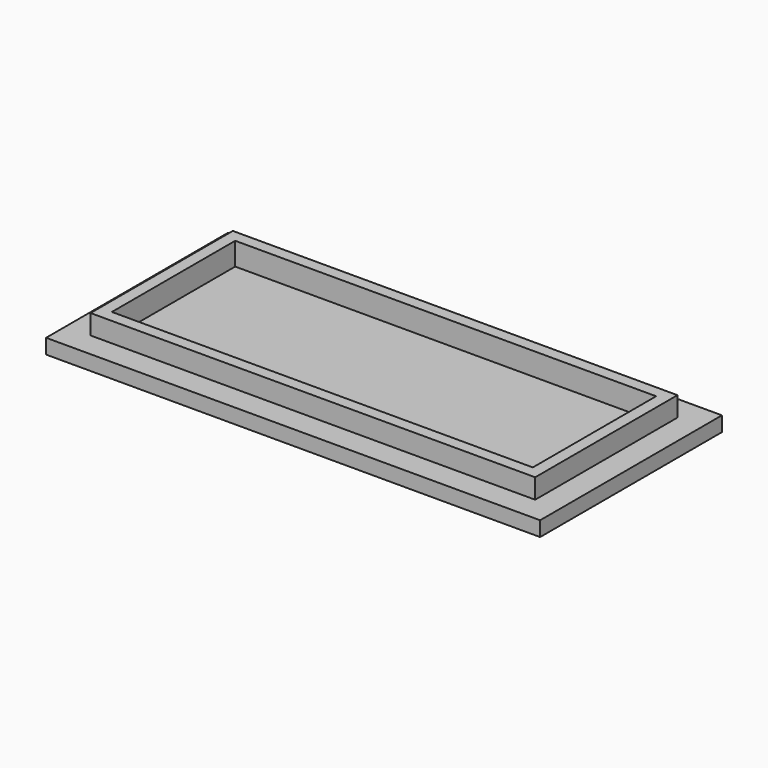
from build123d import *

# Parameters (mm, degrees)
F0_W        = 50
F0_H        = 23
F1_DEPTH    = 1.5
F2_W        = 45
F2_H        = 18
F3_DEPTH    = 2
F4_T        = 1.2
F4_T3_DEPTH = 47.4
F4_T5_DEPTH = 20.4


# Not quite as in the source:
# - a shell that OpenCascade refuses in one call is made with other operations: the cavity is built on its own and cut out


with BuildPart() as f1:
    # F0 (on Top) → F1 (new body)
    with BuildSketch(Plane.XY):
        Rectangle(F0_W, F0_H)
    extrude(amount=F1_DEPTH)

    # F2 (on face) → F3 (join)
    with BuildSketch(Plane.XY.offset(1.5)):
        Rectangle(F2_W, F2_H)
    extrude(amount=F3_DEPTH)

    # F4: shell of thickness 1.2, made by hand


with BuildPart() as f4_core1:
    # F4_t2: copy of F1
    add(f1.part)

    # the walls: a layer under each face that stays
    f4_faces = [f4_core1.faces().sort_by_distance(p)[0] for p in [
        (0, 11.5, 0.75),
        (25, 0, 0.75),
        (-25, 0, 0.75),
        (0, 0, 0),
        (-21.4285714286, -9.8571428571, 1.5),
        (0, -11.5, 0.75),
        (0, 9, 2.5),
        (-22.5, 0, 2.5),
        (0, -9, 2.5),
        (22.5, 0, 2.5),
    ]]
    thicken(f4_faces, amount=-F4_T, mode=Mode.SUBTRACT)

    # F4_s4 → F4_t3 (cut)
    with BuildSketch(Plane.YZ.offset(-23.7)):
        Polygon((9.012, 1.512), (9, 0.3), (7.8, 0.3), (7.8, 1.5), align=None)
        Polygon((-9.012, 1.512), (-9, 0.3), (-7.8, 0.3), (-7.8, 1.5), align=None)
    extrude(amount=F4_T3_DEPTH, mode=Mode.SUBTRACT)

    # F4_s6 → F4_t5 (cut)
    with BuildSketch(Plane.XZ.offset(-10.2)):
        Polygon((-22.512, 1.512), (-22.5, 0.3), (-21.3, 0.3), (-21.3, 1.5), align=None)
        Polygon((22.512, 1.512), (22.5, 0.3), (21.3, 0.3), (21.3, 1.5), align=None)
    extrude(amount=F4_T5_DEPTH, mode=Mode.SUBTRACT)


with BuildPart() as f1_1:
    add(f1.part)

    # what is left inside the walls is the cavity
    f4_cavity = [f4_core1.part.solids().sort_by_distance(p)[0] for p in [
        (0, -2.6, 3.488),
    ]]
    add(f4_cavity, mode=Mode.SUBTRACT)


solid = f1_1.part
